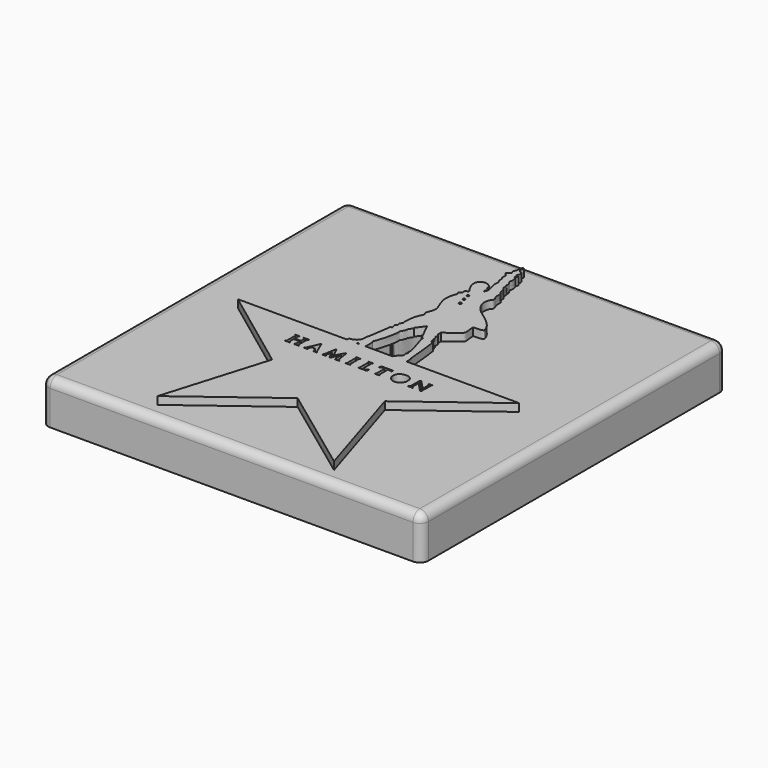
from build123d import *

# Parameters (mm, degrees)
F0_W     = 112.150773406
F0_H     = 112.4793700874
F1_DEPTH = 12.7
F2_R     = 2.54
F0_R     = 0.3681727426
F0_R_2   = 0.3485105907
F0_R_3   = 0.3177347812
F3_DEPTH = 2.286


with BuildPart() as f1:
    # F0 (on Top) → F1 (new body)
    with BuildSketch(Plane.XY):
        with Locations((-19.9486985803, 0.0044340268)):
            Rectangle(F0_W, F0_H)
        with BuildLine():
            Line((-36.7362201214, -20.2893279493), (-61.7272146046, -1.6893827124))
            Line((-61.7272146046, -1.6893827124), (-29.4691417366, -1.6893827124))
            add(Edge.make_bspline(
                [(-29.4691417366, -1.6893827124), (-29.5237013721, -1.4388390749), (-29.6463965163, -0.8754099484), (-28.3983555774, -0.9554241319), (-26.7078402525, 0.2276842475), (-26.9551935497, 1.9249232654), (-26.5510287405, 2.8625786401), (-26.3314076468, 4.5083309506), (-25.9015047243, 7.494346048), (-25.6234984845, 9.4253187999)],
                knots=[0, 0, 0, 0, 0.0894200247, 0.2010901051, 0.3559510971, 0.4960087509, 0.6056512318, 0.7449856409, 1, 1, 1, 1], degree=3))
            add(Edge.make_bspline(
                [(-25.2333423139, 9.5635333242), (-25.3219227435, 9.4874764327), (-25.472710614, 9.4563976163), (-25.6234984845, 9.4253187999)],
                knots=[0.7801649113, 0.7801649113, 0.7801649113, 0.7801649113, 1, 1, 1, 1], degree=3))
            add(Edge.make_bspline(
                [(-25.1598563128, 9.6837207406), (-25.1752593426, 9.6338688339), (-25.2006286539, 9.5947473496), (-25.2333423139, 9.5635333242)],
                knots=[0.9714759624, 0.9714759624, 0.9714759624, 0.9714759624, 0.9789800766, 0.9789800766, 0.9789800766, 0.9789800766], degree=3))
            add(Edge.make_bspline(
                [(-25.2453368157, 11.0025666654), (-25.3321119303, 10.9160826288), (-25.5617885462, 10.6871764389), (-25.107754588, 9.9194596197), (-25.1598563045, 9.6837207675)],
                knots=[0, 0, 0, 0, 0.2605079512, 0.6895131734, 0.6895131734, 0.6895131734, 0.6895131734], degree=3))
            add(Edge.make_bspline(
                [(-22.9490343481, 35.2624803782), (-22.8018357414, 35.1113034083), (-22.540617676, 34.8430253557), (-22.4895259946, 34.2657402758), (-23.0460001446, 34.526176423), (-23.5906009269, 34.1110372145), (-23.2327092542, 33.0681226354), (-24.1035431449, 32.8502167821), (-24.1455210979, 32.1761867134), (-23.6903403339, 31.9969555093), (-24.2741645389, 31.087427418), (-24.607264612, 29.1923440497), (-24.6257458216, 27.534928222), (-23.5218037748, 24.6259469814), (-22.9836414331, 23.5709722175), (-22.952453391, 22.4160750804), (-23.5865090532, 20.5752009755), (-23.9246943644, 20.091176539), (-23.3170598263, 19.5304758984), (-23.5535849601, 18.6516761122), (-24.5950160647, 16.873454437), (-24.7729976776, 13.3684521881), (-24.4989003808, 12.6954615361), (-25.2338553727, 12.2050267632), (-24.7626907381, 11.3691063686), (-25.189514063, 11.2142507799), (-25.2453368157, 11.0025666654)],
                knots=[0, 0, 0, 0, 0.0307314758, 0.0545359554, 0.0802622588, 0.1090081497, 0.1458203396, 0.1785646845, 0.2067190209, 0.2288942713, 0.2654199481, 0.3198613722, 0.371921587, 0.4401794731, 0.482543071, 0.5241536219, 0.5787128626, 0.6062237119, 0.6376563929, 0.6719400889, 0.7295632437, 0.8023925276, 0.8329884951, 0.8649706998, 0.8980080691, 0.9264666099, 0.9264666099, 0.9264666099, 0.9264666099], degree=3))
            add(Edge.make_bspline(
                [(-22.9490343481, 35.2624803782), (-23.139946789, 35.5483260953), (-23.5664430021, 36.1869021639), (-24.1843212935, 37.7463179322), (-24.2473370274, 39.1298976226), (-23.4560503833, 40.1855046325), (-22.0158738609, 40.4813395391), (-21.1345895273, 39.9813063378), (-20.2569942336, 39.4304306948), (-20.3637381443, 38.897921572), (-20.2796970639, 38.2850997483), (-19.8289932326, 38.2755526522), (-19.6463387374, 37.3598565212), (-20.0188424145, 37.4141152424), (-19.9952060808, 36.9277918817), (-19.8662355893, 36.8726857198), (-19.8133550584, 36.8500910699)],
                knots=[0, 0, 0, 0, 0.0865711903, 0.1933990507, 0.2888785835, 0.3793595779, 0.4749403848, 0.5590002659, 0.6382493929, 0.6963700047, 0.7561094623, 0.8062798802, 0.8762223552, 0.9142788001, 0.9648525604, 1, 1, 1, 1], degree=3))
            add(Edge.make_bspline(
                [(-20.9168801994, 45.627435652), (-20.9478766214, 45.2208834106), (-20.9533659654, 44.6259287046), (-20.4849327527, 44.5313410854), (-20.6369049495, 43.1855228646), (-20.0038671401, 42.5986645036), (-20.2482617159, 41.1198147063), (-19.9978500152, 40.3581215802), (-19.7938336586, 39.3522803573), (-19.4744600601, 38.5358663308), (-19.4479877539, 37.4801111999), (-19.6989008341, 37.0474499041), (-19.8133550584, 36.8500910699)],
                knots=[0.0360630283, 0.0360630283, 0.0360630283, 0.0360630283, 0.1242068236, 0.1851782856, 0.2966432502, 0.3917629941, 0.5127643526, 0.6076215214, 0.7103412171, 0.8089702523, 0.912861611, 1, 1, 1, 1], degree=3))
            add(Edge.make_bspline(
                [(-20.8695437759, 46.1448132992), (-20.8868710714, 45.9692925815), (-20.904198367, 45.7937718638), (-20.9168801994, 45.627435652)],
                knots=[0, 0, 0, 0, 0.0360630283, 0.0360630283, 0.0360630283, 0.0360630283], degree=3))
            add(Edge.make_bspline(
                [(-18.347883597, 46.5119630098), (-18.5665247814, 46.567802138), (-19.0423765421, 46.6893306943), (-18.2627145813, 47.1689787625), (-18.2367361184, 47.7493050998), (-19.0725823668, 47.3905741215), (-19.088893013, 48.0398847894), (-18.7304085511, 48.0976478552), (-18.7503885355, 49.4485114254), (-19.0919856996, 49.4405055125), (-19.8176031925, 49.8216608162), (-19.7037560022, 50.1156142091), (-20.3129336884, 49.80698637), (-19.7587928881, 51.1217233446), (-19.7435543422, 51.4120393297), (-20.0107193808, 51.5382141059), (-20.2794145128, 51.4118220515), (-20.5004817284, 50.6496469697), (-20.4362358727, 49.882498514), (-20.8009168457, 49.1893636317), (-20.9273529464, 48.7332131529), (-20.8925448275, 48.2669954972), (-20.6412482291, 48.1561471207), (-20.5147824402, 47.7058883888), (-21.9358148565, 47.3336879099), (-21.6181519328, 46.7525669856), (-20.9801609918, 46.3832501401), (-20.8695437759, 46.1448132992)],
                knots=[0, 0, 0, 0, 0.0376916153, 0.0820322189, 0.1137974968, 0.1561055059, 0.1896032953, 0.2191619444, 0.2766574644, 0.3065577694, 0.3531914623, 0.3742264112, 0.4026228677, 0.4593494332, 0.4892621532, 0.5148329365, 0.5414803994, 0.5880811517, 0.6365811289, 0.6833313589, 0.721149373, 0.7557537263, 0.7824513604, 0.8117225815, 0.8708909914, 0.9059534895, 0.9596486512, 0.9596486512, 0.9596486512, 0.9596486512], degree=3))
            add(Edge.make_bspline(
                [(-10.6186084449, 21.2349332869), (-10.2465425455, 21.2284238876), (-9.4544342281, 21.214565726), (-7.6149963334, 21.4435028641), (-7.7546066038, 21.9755665302), (-8.3391571882, 23.8893715496), (-11.6435767501, 26.7778304182), (-14.0629700087, 28.2270962995), (-15.6854792042, 30.1263664764), (-16.2090457881, 31.5329948027), (-16.5284698213, 32.27210859), (-16.155401142, 34.4002204445), (-15.5027668384, 34.5846284007), (-15.6017769638, 35.5779693835), (-15.8742117791, 36.0210543155), (-16.1304009084, 36.4184531839), (-16.0265131707, 38.1674901169), (-16.2764004031, 38.5351311452), (-16.8721687835, 38.9357832389), (-16.6937824367, 40.2362114298), (-17.2292280837, 40.7266224241), (-17.6365231412, 41.0469906699), (-17.3561192602, 42.0939067716), (-17.659514749, 42.170875727), (-17.8301914046, 42.3491690169), (-17.54351403, 42.8448295654), (-17.7586691842, 43.5126316811), (-18.3019000606, 44.1150281652), (-18.2884014697, 44.4958319827), (-18.0397324808, 45.0119159976), (-18.2280644025, 45.9286958552), (-18.347883597, 46.5119630098)],
                knots=[0, 0, 0, 0, 0.0396143483, 0.08433682, 0.1041713684, 0.1519460453, 0.2258554486, 0.2864297066, 0.3409726353, 0.3825425785, 0.4150064283, 0.4643850722, 0.4905398674, 0.5230436291, 0.548230002, 0.5723701083, 0.6180200404, 0.6412526266, 0.6686294341, 0.7072238622, 0.7358734481, 0.7600779865, 0.7939450096, 0.8106238093, 0.82581542, 0.8504611911, 0.8797997868, 0.9109629421, 0.931131062, 0.9561846945, 1, 1, 1, 1], degree=3))
            add(Edge.make_bspline(
                [(-10.6186084449, 21.2349332869), (-10.603608336, 20.7564123192), (-10.5733991197, 19.7927030843), (-10.2433534529, 18.1499450487), (-10.9858279929, 17.259828738), (-13.2220224996, 15.6233748591), (-14.7604979575, 14.4975138828)],
                knots=[0, 0, 0, 0, 0.216403352, 0.4358218821, 0.611852106, 1, 1, 1, 1], degree=3))
            add(Edge.make_bspline(
                [(-14.7604979575, 14.4975138828), (-14.7604979575, 14.114885591), (-14.7604979575, 13.7322572991), (-14.7604979575, 13.3496290073)],
                knots=[0, 0, 0, 0, 1.1478848755, 1.1478848755, 1.1478848755, 1.1478848755], degree=3))
            add(Edge.make_bspline(
                [(-14.7604979575, 13.3496290073), (-14.6709633377, 13.3205609539), (-14.4511044208, 13.2491821873), (-14.2254039891, 12.5881378504), (-14.5406368419, 12.0748556147), (-14.0358580555, 11.6427740014), (-14.0050283754, 11.1089523301), (-14.0226844223, 10.7298311451), (-13.5725409001, 10.669986686), (-13.9018867308, 10.3380267483), (-13.9797726977, 10.2279725616), (-13.6024465663, 9.3708289172), (-13.2845557848, 9.9440029174), (-12.9462724251, 9.0875406338), (-12.2046987376, 0.9394447277), (-12.1733197621, 0.2789110131), (-11.8637778099, -0.3124650214), (-11.9014828047, -1.1634369089), (-11.9247864932, -1.6893827124)],
                knots=[0, 0, 0, 0, 0.0405911747, 0.0996746479, 0.153531573, 0.2093840106, 0.2640899969, 0.3067246096, 0.3458505858, 0.3879978591, 0.41843724, 0.4802456454, 0.5210262513, 0.5756892974, 0.791696917, 0.856577341, 0.9113571826, 1, 1, 1, 1], degree=3))
            Line((-11.9247864932, -1.6893827124), (21.3132724166, -1.6893827124))
            Line((21.3132724166, -1.6893827124), (-3.4634394106, -20.2893279493))
            Line((-3.4634394106, -20.2893279493), (6.1069312505, -51.013097167))
            Line((6.1069312505, -51.013097167), (-20.1285295188, -31.6414646804))
            Line((-20.1285295188, -31.6414646804), (-45.9681414068, -51.013097167))
            Line((-45.9681414068, -51.013097167), (-36.7362201214, -20.2893279493))
        make_face(mode=Mode.SUBTRACT)
        with BuildLine():
            add(Edge.make_bspline(
                [(-25.1598563128, 9.6837207406), (-25.1752593426, 9.6338688339), (-25.2006286539, 9.5947473496), (-25.2333423139, 9.5635333242)],
                knots=[0.9714759624, 0.9714759624, 0.9714759624, 0.9714759624, 0.9789800766, 0.9789800766, 0.9789800766, 0.9789800766], degree=3))
            add(Edge.make_bspline(
                [(-25.1598563045, 9.6837207675), (-25.1708657536, 9.6339075356), (-25.1968150701, 9.594896331), (-25.2333423139, 9.5635333242)],
                knots=[0.6895131734, 0.6895131734, 0.6895131734, 0.6895131734, 0.7801649113, 0.7801649113, 0.7801649113, 0.7801649113], degree=3))
        make_face()
    extrude(amount=-F1_DEPTH)

    # F2
    f2_edges = [f1.edges().sort_by_distance(p)[0] for p in [
        (-76.024085, 0.004434, 0),
        (-19.948699, -56.235251, 0),
        (36.126688, 0.004434, 0),
        (-19.948699, 56.244119, 0),
        (-76.024085, 56.244119, -6.35),
        (36.126688, -56.235251, -6.35),
        (36.126688, 56.244119, -6.35),
        (-76.024085, -56.235251, -6.35),
    ]]
    fillet(f2_edges, radius=F2_R)


with BuildPart() as f3:
    # F0 (on Top) → F3 (new body)
    with BuildSketch(Plane.XY):
        Polygon((-29.4691417366, -1.6893827124), (-61.7272146046, -1.6893827124), (-36.7362201214, -20.2893279493), (-45.9681414068, -51.013097167), (-20.1285295188, -31.6414646804), (6.1069312505, -51.013097167), (-3.4634394106, -20.2893279493), (21.3132724166, -1.6893827124), (-11.9247864932, -1.6893827124), (-15.9918069839, -1.6893827124), (-24.053927511, -1.6893827124), (-26.0321982205, -1.6893827124), (-26.5392046422, -1.6893827124), align=None)
        Polygon((-40.0256514549, -7.5422911905), (-40.4652655125, -7.2247912176), (-38.9876700938, -7.2247912176), (-39.2495194952, -7.421096425), (-39.2495194952, -8.7878685445), (-37.4245941639, -8.7878685445), (-37.4245941639, -7.5388336554), (-37.8803871572, -7.2247912176), (-36.2271368504, -7.2247912176), (-36.617346108, -7.610714063), (-36.617346108, -10.7172913849), (-36.1963324249, -11.0836373642), (-37.818774581, -11.0836373642), (-37.4593734741, -10.7172913849), (-37.4593734741, -9.2172604054), (-39.2495194952, -9.2172604054), (-39.2495194952, -10.7323806733), (-38.7922860682, -11.0836373642), (-40.4652655125, -11.0836373642), (-40.0256514549, -10.7172913849), align=None, mode=Mode.SUBTRACT)
        Polygon((-33.7780527771, -10.756380856), (-33.4943346679, -11.0916616395), (-34.9104516208, -11.0916616395), (-34.4096310437, -10.7462676242), (-32.8553542495, -7.1887043305), (-32.6916128397, -7.1887043305), (-31.1201103032, -10.8286002651), (-30.7292062789, -11.0916616395), (-31.8619273603, -11.0916616395), (-32.4326083064, -9.8269563168), (-33.4943346679, -9.8269563168), align=None, mode=Mode.SUBTRACT)
        Polygon((-28.2085649669, -11.1190462485), (-29.4778887182, -11.1190462485), (-29.0806852281, -10.7391122729), (-28.4848809242, -7.2160884738), (-28.2517392188, -7.2160884738), (-26.9565097988, -9.8756263033), (-25.4673454911, -7.164278999), (-25.3115762025, -7.164278999), (-24.7330404818, -10.7100671157), (-24.193353951, -11.1276805401), (-25.5749318749, -11.1276805401), (-25.7864929736, -8.6549706757), (-26.874486357, -11.1276805401), (-27.1767061204, -11.1276805401), (-28.2517392188, -8.7444586679), (-28.4503418952, -10.8168255538), align=None, mode=Mode.SUBTRACT)
        Polygon((-20.8046101034, -11.1276805401), (-22.5194729865, -11.1276805401), (-22.1806075424, -10.6879072264), (-22.1806075424, -7.5148972683), (-22.5092042238, -7.2479126975), (-20.9791772068, -7.2479126975), (-21.2872363627, -7.6381210238), (-21.2872363627, -10.759787634), align=None, mode=Mode.SUBTRACT)
        with BuildLine():
            Line((-18.5136832297, -7.4280803092), (-18.8331697136, -7.2175106034))
            Line((-18.8331697136, -7.2175106034), (-17.2793101519, -7.2175106034))
            Line((-17.2793101519, -7.2175106034), (-17.6154654473, -7.4356948026))
            Line((-17.6154654473, -7.4356948026), (-17.6154654473, -10.4060871527))
            Line((-17.6154654473, -10.4060871527), (-17.6085237545, -10.622094177))
            ThreePointArc((-17.6085237545, -10.622094177), (-17.5923960548, -10.6593838903), (-17.555142433, -10.6755947843))
            add(Edge.make_bspline(
                [(-16.1923579872, -10.121867992), (-16.3024780791, -10.2929745357), (-16.490348645, -10.584891139), (-16.7619889875, -10.7002475533), (-17.2457192524, -10.6862299666), (-17.555142433, -10.6755947843)],
                knots=[0, 0, 0, 0, 0.3382231569, 0.5770261788, 0.9776933849, 0.9776933849, 0.9776933849, 0.9776933849], degree=3))
            add(Edge.make_bspline(
                [(-16.415219754, -11.0537018627), (-16.359229354, -11.0459337224), (-16.226757673, -11.0275545251), (-16.1333393742, -10.6854865133), (-16.1706334808, -10.3293336291), (-16.1923579872, -10.121867992)],
                knots=[0, 0, 0, 0, 0.2340860987, 0.5538409976, 1, 1, 1, 1], degree=3))
            Line((-16.415219754, -11.0537018627), (-18.8331697136, -11.0537018627))
            Line((-18.8331697136, -11.0537018627), (-18.5136832297, -10.6910374016))
            Line((-18.5136832297, -10.6910374016), (-18.5136832297, -7.4280803092))
        make_face(mode=Mode.SUBTRACT)
        with BuildLine():
            Line((-15.0807779282, -7.9221175984), (-14.9041190743, -7.1939183399))
            Line((-14.9041190743, -7.1939183399), (-11.5278875455, -7.1939183399))
            Line((-11.5278875455, -7.1939183399), (-11.5278875455, -8.0487700179))
            add(Edge.make_bspline(
                [(-11.5278875455, -8.0487700179), (-11.5433357335, -8.0268931558), (-11.5842795953, -7.9689107426), (-11.6508747214, -7.8265296344), (-11.7067676038, -7.755109109)],
                knots=[0, 0, 0, 0, 0.1864501849, 0.4941673807, 0.4941673807, 0.4941673807, 0.4941673807], degree=3))
            add(Edge.make_bspline(
                [(-11.7067676038, -7.755109109), (-11.7599063532, -7.6872078442), (-11.874326853, -7.5967481357), (-11.9660361084, -7.5988073284), (-12.0047042146, -7.5996755622)],
                knots=[0.4941673807, 0.4941673807, 0.4941673807, 0.4941673807, 0.7867217503, 1, 1, 1, 1], degree=3))
            Line((-12.0047042146, -7.5996755622), (-12.755936943, -7.5996755622))
            Line((-12.755936943, -7.5996755622), (-12.755936943, -10.8269555494))
            Line((-12.755936943, -10.8269555494), (-12.3587334529, -11.0341925174))
            Line((-12.3587334529, -11.0341925174), (-13.9475483447, -11.0341925174))
            Line((-13.9475483447, -11.0341925174), (-13.6539638042, -10.801050812))
            Line((-13.6539638042, -10.801050812), (-13.6539638042, -7.5996755622))
            Line((-13.6539638042, -7.5996755622), (-14.6404961124, -7.5996755622))
            Line((-14.6404961124, -7.5996755622), (-15.0807779282, -7.9221175984))
        make_face(mode=Mode.SUBTRACT)
        with BuildLine():
            add(Edge.make_bspline(
                [(-9.9246390164, -9.5042390749), (-9.9889846759, -9.1853929712), (-10.0735427643, -8.3701330766), (-8.9447383122, -7.081842496), (-7.075462484, -7.1046648861), (-6.6941387365, -7.3184325157), (-5.7626662195, -7.8300610845), (-5.5757053849, -9.4046076741), (-6.0340100651, -10.5022288737), (-7.0370483695, -11.3757346143), (-8.8056540963, -11.2782214727), (-9.6950125829, -10.3304409953), (-9.8672990139, -9.7883706931), (-9.9246390164, -9.5042390749)],
                knots=[0, 0, 0, 0, 0.0861005374, 0.1914415764, 0.3012806293, 0.3571649442, 0.4380250942, 0.5399885089, 0.6306555154, 0.7237094275, 0.8310412643, 0.9232736899, 1, 1, 1, 1], degree=3))
        make_face(mode=Mode.SUBTRACT)
        with BuildLine():
            ThreePointArc((-3.5721734927, -10.7660449712), (-3.5582374808, -10.7472784259), (-3.5532980692, -10.7244311534))
            Line((-3.5532980692, -10.7244311534), (-3.5532980692, -7.2171073407))
            Line((-3.5532980692, -7.2171073407), (-3.1425524503, -7.2171073407))
            Line((-3.1425524503, -7.2171073407), (-0.5651239771, -9.9382968619))
            Line((-0.5651239771, -9.9382968619), (-0.5651239771, -7.5559723191))
            Line((-0.5651239771, -7.5559723191), (-1.0374814738, -7.2376444004))
            Line((-1.0374814738, -7.2376444004), (0.3282474936, -7.2376444004))
            Line((0.3282474936, -7.2376444004), (0, -7.5866607949))
            Line((0, -7.5866607949), (-0.0699376687, -11.1516881734))
            Line((-0.0699376687, -11.1516881734), (-0.3909707884, -11.1661935225))
            Line((-0.3909707884, -11.1661935225), (-3.0106524937, -8.3852373064))
            Line((-3.0106524937, -8.3852373064), (-3.0106524937, -10.7291993712))
            ThreePointArc((-3.0106524937, -10.7291993712), (-3.0038159244, -10.7558361832), (-2.9849962854, -10.7758881063))
            Line((-2.9849962854, -10.7758881063), (-2.4733366445, -11.1008603126))
            Line((-2.4733366445, -11.1008603126), (-3.9545856416, -11.1008603126))
            Line((-3.9545856416, -11.1008603126), (-3.5721734927, -10.7660449712))
        make_face(mode=Mode.SUBTRACT)
        with BuildLine():
            add(Edge.make_bspline(
                [(-29.4691417366, -1.6893827124), (-29.5237013721, -1.4388390749), (-29.6463965163, -0.8754099484), (-28.3983555774, -0.9554241319), (-26.7078402525, 0.2276842475), (-26.9551935497, 1.9249232654), (-26.5510287405, 2.8625786401), (-26.3314076468, 4.5083309506), (-25.9015047243, 7.494346048), (-25.6234984845, 9.4253187999)],
                knots=[0, 0, 0, 0, 0.0894200247, 0.2010901051, 0.3559510971, 0.4960087509, 0.6056512318, 0.7449856409, 1, 1, 1, 1], degree=3))
            Line((-29.4691417366, -1.6893827124), (-26.5392046422, -1.6893827124))
            Line((-26.5392046422, -1.6893827124), (-26.5289358795, -1.4415598707))
            Line((-26.5289358795, -1.4415598707), (-26.1295708957, -1.4581079186))
            Line((-26.1295708957, -1.4581079186), (-26.0321982205, -1.6893827124))
            Line((-26.0321982205, -1.6893827124), (-24.053927511, -1.6893827124))
            Line((-24.053927511, -1.6893827124), (-24.053927511, 0.8218600415))
            add(Edge.make_bspline(
                [(-21.1157724261, 12.5192441046), (-21.0780867635, 12.3971107124), (-20.9735096341, 12.0581924433), (-22.0265415448, 10.9737253663), (-21.6446727931, 10.4983963575), (-22.3108366062, 9.865685903), (-22.056872514, 9.4782131102), (-22.7221047305, 9.1599672036), (-22.1995061559, 8.0840928477), (-23.9410529938, 1.6342335308), (-24.438002766, 1.4101826494), (-24.1908262428, 1.0315601403), (-24.053927511, 0.8218600415)],
                knots=[0, 0, 0, 0, 0.0676749399, 0.1877969087, 0.2581596624, 0.3483193009, 0.4078375091, 0.4786169858, 0.5879963721, 0.8540293142, 0.9191541271, 1, 1, 1, 1], degree=3))
            Line((-21.1157724261, 12.5192441046), (-19.2606505007, 15.0392493233))
            Line((-19.2606505007, 15.0392493233), (-16.6109707206, 9.7455587238))
            add(Edge.make_bspline(
                [(-15.9918069839, -1.6893827124), (-16.0252978829, -1.5998634295), (-16.1367659505, -1.3019155755), (-14.7158356306, -0.201382184), (-14.2887593985, 0.1877216705), (-14.6606368373, 1.3546729471), (-14.3041571084, 1.5507152158), (-14.2987769787, 2.0923980308), (-14.6740799981, 1.8262645585), (-13.9952852464, 3.081836288), (-16.5827953232, 9.4515542281), (-16.1569471987, 9.8153962133), (-16.4324523843, 9.6835882983), (-16.6109707206, 9.7455587238)],
                knots=[0, 0, 0, 0, 0.0454512894, 0.1512759453, 0.2146236619, 0.2970134763, 0.3465876708, 0.3956429731, 0.4281281446, 0.5067740617, 0.7211580995, 0.7551998499, 0.8044892445, 0.8044892445, 0.8044892445, 0.8044892445], degree=3))
            Line((-15.9918069839, -1.6893827124), (-11.9247864932, -1.6893827124))
            add(Edge.make_bspline(
                [(-14.7604979575, 13.3496290073), (-14.6709633377, 13.3205609539), (-14.4511044208, 13.2491821873), (-14.2254039891, 12.5881378504), (-14.5406368419, 12.0748556147), (-14.0358580555, 11.6427740014), (-14.0050283754, 11.1089523301), (-14.0226844223, 10.7298311451), (-13.5725409001, 10.669986686), (-13.9018867308, 10.3380267483), (-13.9797726977, 10.2279725616), (-13.6024465663, 9.3708289172), (-13.2845557848, 9.9440029174), (-12.9462724251, 9.0875406338), (-12.2046987376, 0.9394447277), (-12.1733197621, 0.2789110131), (-11.8637778099, -0.3124650214), (-11.9014828047, -1.1634369089), (-11.9247864932, -1.6893827124)],
                knots=[0, 0, 0, 0, 0.0405911747, 0.0996746479, 0.153531573, 0.2093840106, 0.2640899969, 0.3067246096, 0.3458505858, 0.3879978591, 0.41843724, 0.4802456454, 0.5210262513, 0.5756892974, 0.791696917, 0.856577341, 0.9113571826, 1, 1, 1, 1], degree=3))
            add(Edge.make_bspline(
                [(-14.7604979575, 14.4975138828), (-14.7604979575, 14.114885591), (-14.7604979575, 13.7322572991), (-14.7604979575, 13.3496290073)],
                knots=[0, 0, 0, 0, 1.1478848755, 1.1478848755, 1.1478848755, 1.1478848755], degree=3))
            add(Edge.make_bspline(
                [(-10.6186084449, 21.2349332869), (-10.603608336, 20.7564123192), (-10.5733991197, 19.7927030843), (-10.2433534529, 18.1499450487), (-10.9858279929, 17.259828738), (-13.2220224996, 15.6233748591), (-14.7604979575, 14.4975138828)],
                knots=[0, 0, 0, 0, 0.216403352, 0.4358218821, 0.611852106, 1, 1, 1, 1], degree=3))
            add(Edge.make_bspline(
                [(-10.6186084449, 21.2349332869), (-10.2465425455, 21.2284238876), (-9.4544342281, 21.214565726), (-7.6149963334, 21.4435028641), (-7.7546066038, 21.9755665302), (-8.3391571882, 23.8893715496), (-11.6435767501, 26.7778304182), (-14.0629700087, 28.2270962995), (-15.6854792042, 30.1263664764), (-16.2090457881, 31.5329948027), (-16.5284698213, 32.27210859), (-16.155401142, 34.4002204445), (-15.5027668384, 34.5846284007), (-15.6017769638, 35.5779693835), (-15.8742117791, 36.0210543155), (-16.1304009084, 36.4184531839), (-16.0265131707, 38.1674901169), (-16.2764004031, 38.5351311452), (-16.8721687835, 38.9357832389), (-16.6937824367, 40.2362114298), (-17.2292280837, 40.7266224241), (-17.6365231412, 41.0469906699), (-17.3561192602, 42.0939067716), (-17.659514749, 42.170875727), (-17.8301914046, 42.3491690169), (-17.54351403, 42.8448295654), (-17.7586691842, 43.5126316811), (-18.3019000606, 44.1150281652), (-18.2884014697, 44.4958319827), (-18.0397324808, 45.0119159976), (-18.2280644025, 45.9286958552), (-18.347883597, 46.5119630098)],
                knots=[0, 0, 0, 0, 0.0396143483, 0.08433682, 0.1041713684, 0.1519460453, 0.2258554486, 0.2864297066, 0.3409726353, 0.3825425785, 0.4150064283, 0.4643850722, 0.4905398674, 0.5230436291, 0.548230002, 0.5723701083, 0.6180200404, 0.6412526266, 0.6686294341, 0.7072238622, 0.7358734481, 0.7600779865, 0.7939450096, 0.8106238093, 0.82581542, 0.8504611911, 0.8797997868, 0.9109629421, 0.931131062, 0.9561846945, 1, 1, 1, 1], degree=3))
            add(Edge.make_bspline(
                [(-18.347883597, 46.5119630098), (-18.5665247814, 46.567802138), (-19.0423765421, 46.6893306943), (-18.2627145813, 47.1689787625), (-18.2367361184, 47.7493050998), (-19.0725823668, 47.3905741215), (-19.088893013, 48.0398847894), (-18.7304085511, 48.0976478552), (-18.7503885355, 49.4485114254), (-19.0919856996, 49.4405055125), (-19.8176031925, 49.8216608162), (-19.7037560022, 50.1156142091), (-20.3129336884, 49.80698637), (-19.7587928881, 51.1217233446), (-19.7435543422, 51.4120393297), (-20.0107193808, 51.5382141059), (-20.2794145128, 51.4118220515), (-20.5004817284, 50.6496469697), (-20.4362358727, 49.882498514), (-20.8009168457, 49.1893636317), (-20.9273529464, 48.7332131529), (-20.8925448275, 48.2669954972), (-20.6412482291, 48.1561471207), (-20.5147824402, 47.7058883888), (-21.9358148565, 47.3336879099), (-21.6181519328, 46.7525669856), (-20.9801609918, 46.3832501401), (-20.8695437759, 46.1448132992)],
                knots=[0, 0, 0, 0, 0.0376916153, 0.0820322189, 0.1137974968, 0.1561055059, 0.1896032953, 0.2191619444, 0.2766574644, 0.3065577694, 0.3531914623, 0.3742264112, 0.4026228677, 0.4593494332, 0.4892621532, 0.5148329365, 0.5414803994, 0.5880811517, 0.6365811289, 0.6833313589, 0.721149373, 0.7557537263, 0.7824513604, 0.8117225815, 0.8708909914, 0.9059534895, 0.9596486512, 0.9596486512, 0.9596486512, 0.9596486512], degree=3))
            add(Edge.make_bspline(
                [(-20.8695437759, 46.1448132992), (-20.7918986231, 45.977448167), (-20.8499157433, 45.802685843), (-20.9168801994, 45.627435652)],
                knots=[0.9596486512, 0.9596486512, 0.9596486512, 0.9596486512, 0.9973387069, 0.9973387069, 0.9973387069, 0.9973387069], degree=3))
            add(Edge.make_bspline(
                [(-20.9168801994, 45.627435652), (-20.9478766214, 45.2208834106), (-20.9533659654, 44.6259287046), (-20.4849327527, 44.5313410854), (-20.6369049495, 43.1855228646), (-20.0038671401, 42.5986645036), (-20.2482617159, 41.1198147063), (-19.9978500152, 40.3581215802), (-19.7938336586, 39.3522803573), (-19.4744600601, 38.5358663308), (-19.4479877539, 37.4801111999), (-19.6989008341, 37.0474499041), (-19.8133550584, 36.8500910699)],
                knots=[0.0360630283, 0.0360630283, 0.0360630283, 0.0360630283, 0.1242068236, 0.1851782856, 0.2966432502, 0.3917629941, 0.5127643526, 0.6076215214, 0.7103412171, 0.8089702523, 0.912861611, 1, 1, 1, 1], degree=3))
            add(Edge.make_bspline(
                [(-22.9490343481, 35.2624803782), (-23.139946789, 35.5483260953), (-23.5664430021, 36.1869021639), (-24.1843212935, 37.7463179322), (-24.2473370274, 39.1298976226), (-23.4560503833, 40.1855046325), (-22.0158738609, 40.4813395391), (-21.1345895273, 39.9813063378), (-20.2569942336, 39.4304306948), (-20.3637381443, 38.897921572), (-20.2796970639, 38.2850997483), (-19.8289932326, 38.2755526522), (-19.6463387374, 37.3598565212), (-20.0188424145, 37.4141152424), (-19.9952060808, 36.9277918817), (-19.8662355893, 36.8726857198), (-19.8133550584, 36.8500910699)],
                knots=[0, 0, 0, 0, 0.0865711903, 0.1933990507, 0.2888785835, 0.3793595779, 0.4749403848, 0.5590002659, 0.6382493929, 0.6963700047, 0.7561094623, 0.8062798802, 0.8762223552, 0.9142788001, 0.9648525604, 1, 1, 1, 1], degree=3))
            add(Edge.make_bspline(
                [(-22.9490343481, 35.2624803782), (-22.8018357414, 35.1113034083), (-22.540617676, 34.8430253557), (-22.4895259946, 34.2657402758), (-23.0460001446, 34.526176423), (-23.5906009269, 34.1110372145), (-23.2327092542, 33.0681226354), (-24.1035431449, 32.8502167821), (-24.1455210979, 32.1761867134), (-23.6903403339, 31.9969555093), (-24.2741645389, 31.087427418), (-24.607264612, 29.1923440497), (-24.6257458216, 27.534928222), (-23.5218037748, 24.6259469814), (-22.9836414331, 23.5709722175), (-22.952453391, 22.4160750804), (-23.5865090532, 20.5752009755), (-23.9246943644, 20.091176539), (-23.3170598263, 19.5304758984), (-23.5535849601, 18.6516761122), (-24.5950160647, 16.873454437), (-24.7729976776, 13.3684521881), (-24.4989003808, 12.6954615361), (-25.2338553727, 12.2050267632), (-24.7626907381, 11.3691063686), (-25.189514063, 11.2142507799), (-25.2453368157, 11.0025666654)],
                knots=[0, 0, 0, 0, 0.0307314758, 0.0545359554, 0.0802622588, 0.1090081497, 0.1458203396, 0.1785646845, 0.2067190209, 0.2288942713, 0.2654199481, 0.3198613722, 0.371921587, 0.4401794731, 0.482543071, 0.5241536219, 0.5787128626, 0.6062237119, 0.6376563929, 0.6719400889, 0.7295632437, 0.8023925276, 0.8329884951, 0.8649706998, 0.8980080691, 0.9264666099, 0.9264666099, 0.9264666099, 0.9264666099], degree=3))
            add(Edge.make_bspline(
                [(-25.2453368157, 11.0025666654), (-25.3336247534, 10.6677721057), (-25.0674696224, 9.9827303626), (-25.1598563045, 9.6837207675)],
                knots=[0.9264666099, 0.9264666099, 0.9264666099, 0.9264666099, 0.9714759611, 0.9714759611, 0.9714759611, 0.9714759611], degree=3))
            add(Edge.make_bspline(
                [(-25.1598563045, 9.6837207675), (-25.1708657536, 9.6339075356), (-25.1968150701, 9.594896331), (-25.2333423139, 9.5635333242)],
                knots=[0.6895131734, 0.6895131734, 0.6895131734, 0.6895131734, 0.7801649113, 0.7801649113, 0.7801649113, 0.7801649113], degree=3))
            add(Edge.make_bspline(
                [(-25.2333423139, 9.5635333242), (-25.3249771969, 9.4760990975), (-25.4742378407, 9.4507089487), (-25.6234984845, 9.4253187999)],
                knots=[0.9789800766, 0.9789800766, 0.9789800766, 0.9789800766, 1, 1, 1, 1], degree=3))
        make_face()
        with Locations((-20.4431116581, 28.7776254117)):
            Circle(F0_R, mode=Mode.SUBTRACT)
        with Locations((-20.9871064872, 30.8586247265)):
            Circle(F0_R_2, mode=Mode.SUBTRACT)
        with Locations((-21.3929433376, 32.8187383711)):
            Circle(F0_R_3, mode=Mode.SUBTRACT)
        with BuildLine():
            add(Edge.make_bspline(
                [(-25.2333423139, 9.5635333242), (-25.3219227435, 9.4874764327), (-25.472710614, 9.4563976163), (-25.6234984845, 9.4253187999)],
                knots=[0.7801649113, 0.7801649113, 0.7801649113, 0.7801649113, 1, 1, 1, 1], degree=3))
            add(Edge.make_bspline(
                [(-25.2333423139, 9.5635333242), (-25.3249771969, 9.4760990975), (-25.4742378407, 9.4507089487), (-25.6234984845, 9.4253187999)],
                knots=[0.9789800766, 0.9789800766, 0.9789800766, 0.9789800766, 1, 1, 1, 1], degree=3))
        make_face()
        with BuildLine():
            add(Edge.make_bspline(
                [(-25.2453368157, 11.0025666654), (-25.3321119303, 10.9160826288), (-25.5617885462, 10.6871764389), (-25.107754588, 9.9194596197), (-25.1598563045, 9.6837207675)],
                knots=[0, 0, 0, 0, 0.2605079512, 0.6895131734, 0.6895131734, 0.6895131734, 0.6895131734], degree=3))
            add(Edge.make_bspline(
                [(-25.2453368157, 11.0025666654), (-25.3336247534, 10.6677721057), (-25.0674696224, 9.9827303626), (-25.1598563045, 9.6837207675)],
                knots=[0.9264666099, 0.9264666099, 0.9264666099, 0.9264666099, 0.9714759611, 0.9714759611, 0.9714759611, 0.9714759611], degree=3))
        make_face()
        with BuildLine():
            add(Edge.make_bspline(
                [(-20.8695437759, 46.1448132992), (-20.8868710714, 45.9692925815), (-20.904198367, 45.7937718638), (-20.9168801994, 45.627435652)],
                knots=[0, 0, 0, 0, 0.0360630283, 0.0360630283, 0.0360630283, 0.0360630283], degree=3))
            add(Edge.make_bspline(
                [(-20.8695437759, 46.1448132992), (-20.7918986231, 45.977448167), (-20.8499157433, 45.802685843), (-20.9168801994, 45.627435652)],
                knots=[0.9596486512, 0.9596486512, 0.9596486512, 0.9596486512, 0.9973387069, 0.9973387069, 0.9973387069, 0.9973387069], degree=3))
        make_face()
        with BuildLine():
            add(Edge.make_bspline(
                [(-11.5278875455, -8.0487700179), (-11.5433357335, -8.0268931558), (-11.5842795953, -7.9689107426), (-11.6508747214, -7.8265296344), (-11.7067676038, -7.755109109)],
                knots=[0, 0, 0, 0, 0.1864501849, 0.4941673807, 0.4941673807, 0.4941673807, 0.4941673807], degree=3))
            add(Edge.make_bspline(
                [(-11.7067676038, -7.755109109), (-11.687146886, -7.7756315861), (-11.6428812087, -7.8219316939), (-11.5691400553, -7.9469383891), (-11.5410188782, -8.0163553843), (-11.5278875455, -8.0487700179)],
                knots=[0, 0, 0, 0, 0.2979379914, 0.6721684264, 1, 1, 1, 1], degree=3))
        make_face()
    extrude(amount=F3_DEPTH)


solid = Compound([f1.part, f3.part])
